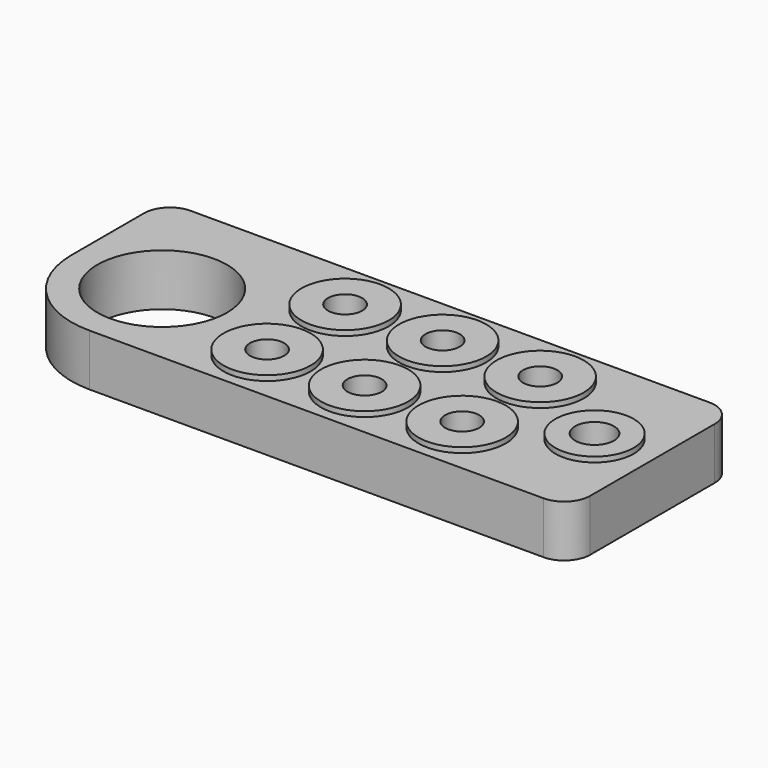
from build123d import *

# Parameters (mm, degrees)
F0_R         = 12.5
F1_DEPTH     = 10
F2_R         = 8.4
F2_R_2       = 3.3
F2_R_3       = 7.55
F2_R_4       = 3.75
F3_DEPTH     = 1
F4_DEPTH     = 9
F5_TEXT_SIZE = 5.5555555556
F6_DEPTH     = 1


# Not quite as in the source:
# - Text() gives the source's letters only with a copy of the font that has no kerning and outlines rounded to 1/6400 em; it was checked with that copy


with BuildPart() as f1:
    # F0 (on Top) → F1 (new body)
    with BuildSketch(Plane.XY):
        with BuildLine():
            ThreePointArc((0, 17.5), (5.1256313292, 5.1256313292), (17.5, 0))
            Line((17.5, 0), (105, 0))
            ThreePointArc((105, 0), (108.5355339059, 1.4644660941), (110, 5))
            Line((110, 5), (110, 35))
            ThreePointArc((110, 35), (108.5355339059, 38.5355339059), (105, 40))
            Line((105, 40), (5, 40))
            ThreePointArc((5, 40), (1.4644660941, 38.5355339059), (0, 35))
            Line((0, 35), (0, 17.5))
        make_face()
        with Locations((17.5, 17.5)):
            Circle(F0_R, mode=Mode.SUBTRACT)
    extrude(amount=F1_DEPTH)

    # F2 (on face) → F3 (join)
    with BuildSketch(Plane.XY.offset(10)):
        with Locations((43.4, 29.2)):
            Circle(F2_R)
        with Locations((43.4, 29.2)):
            Circle(F2_R_2, mode=Mode.SUBTRACT)
        with Locations((62.2, 29.2)):
            Circle(F2_R)
        with Locations((62.2, 29.2)):
            Circle(F2_R_2, mode=Mode.SUBTRACT)
        with Locations((62.2, 10.4)):
            Circle(F2_R)
        with Locations((62.2, 10.4)):
            Circle(F2_R_2, mode=Mode.SUBTRACT)
        with Locations((43.4, 10.4)):
            Circle(F2_R)
        with Locations((43.4, 10.4)):
            Circle(F2_R_2, mode=Mode.SUBTRACT)
        with Locations((81, 10.4)):
            Circle(F2_R)
        with Locations((81, 10.4)):
            Circle(F2_R_2, mode=Mode.SUBTRACT)
        with Locations((81, 29.2)):
            Circle(F2_R)
        with Locations((81, 29.2)):
            Circle(F2_R_2, mode=Mode.SUBTRACT)
        with Locations((99, 19.8)):
            Circle(F2_R_3)
        with Locations((99, 19.8)):
            Circle(F2_R_4, mode=Mode.SUBTRACT)
    extrude(amount=F3_DEPTH)

    # F2 (on face) → F4 (cut)
    with BuildSketch(Plane.XY.offset(10)):
        with Locations((99, 19.8)):
            Circle(F2_R_4)
        with Locations((81, 29.2)):
            Circle(F2_R_2)
        with Locations((81, 10.4)):
            Circle(F2_R_2)
        with Locations((62.2, 10.4)):
            Circle(F2_R_2)
        with Locations((62.2, 29.2)):
            Circle(F2_R_2)
        with Locations((43.4, 29.2)):
            Circle(F2_R_2)
        with Locations((43.4, 10.4)):
            Circle(F2_R_2)
    extrude(amount=-F4_DEPTH, mode=Mode.SUBTRACT)

    # F5 (on face) → F6 (cut)
    with BuildSketch(Plane(origin=(0, 0, 0), x_dir=(1, 0, 0), z_dir=(0, 0, -1))):
        with Locations((30, -9)):
            Text('812', F5_TEXT_SIZE, font='Open Sans', text_align=(TextAlign.LEFT, TextAlign.BOTTOM))
    extrude(amount=-F6_DEPTH, mode=Mode.SUBTRACT)


solid = f1.part
